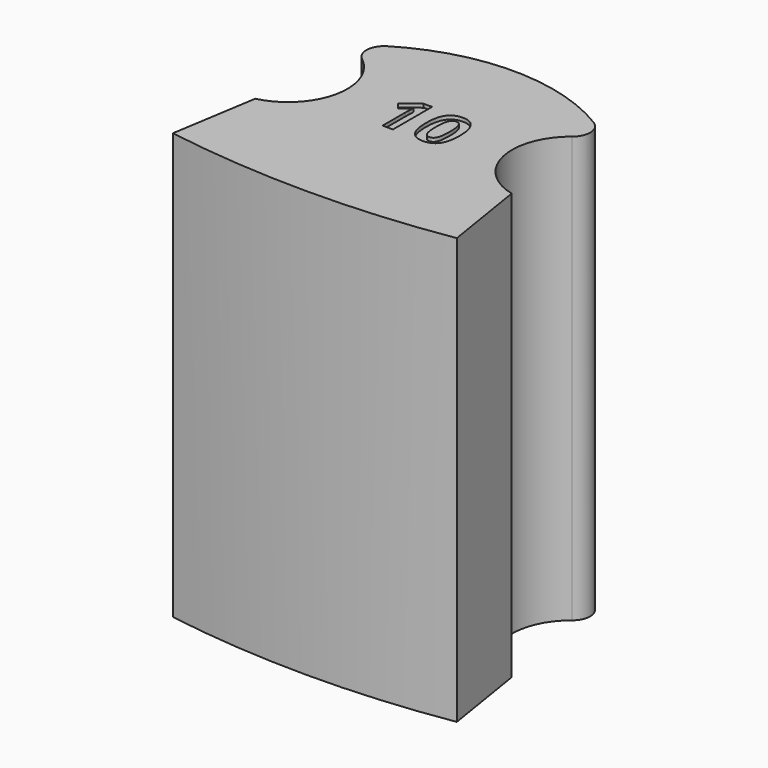
from build123d import *

# Parameters (mm, degrees)
F1_DEPTH     = 120
F2_TEXT_SIZE = 19.2989440014
F3_DEPTH     = 1


# Not quite as in the source:
# - Text() gives the source's letters only with a copy of the font that has no kerning and outlines rounded to 1/6400 em; it was checked with that copy


with BuildPart() as f1:
    # F0 (on Top) → F1 (new body)
    with BuildSketch(Plane.XY):
        with BuildLine():
            Line((3.8687128108, 24.1569802165), (0, 0))
            ThreePointArc((0, 0), (40, -3.1820662963), (80, 0))
            Line((80, 0), (76.1312871892, 24.1569802165))
            ThreePointArc((76.1312871892, 24.1569802165), (63.5975554576, 36.8458138953), (69.5972800683, 53.6417728094))
            ThreePointArc((69.5972800683, 53.6417728094), (71.4969098635, 57.8715436357), (69.1043731597, 61.843359684))
            ThreePointArc((69.1043731597, 61.843359684), (40, 70), (10.8956268403, 61.843359684))
            ThreePointArc((10.8956268403, 61.843359684), (8.5030901365, 57.8715436357), (10.4027199317, 53.6417728094))
            ThreePointArc((10.4027199317, 53.6417728094), (16.4024445424, 36.8458138953), (3.8687128108, 24.1569802165))
        make_face()
    extrude(amount=F1_DEPTH)

    # F2 (on face) → F3 (cut)
    with BuildSketch(Plane.XY.offset(120)):
        with Locations((28.7025791092, 31.6558778286)):
            Text('10', F2_TEXT_SIZE, font='Open Sans', font_style=FontStyle.BOLD, text_align=(TextAlign.LEFT, TextAlign.BOTTOM))
    extrude(amount=-F3_DEPTH, mode=Mode.SUBTRACT)


solid = f1.part
